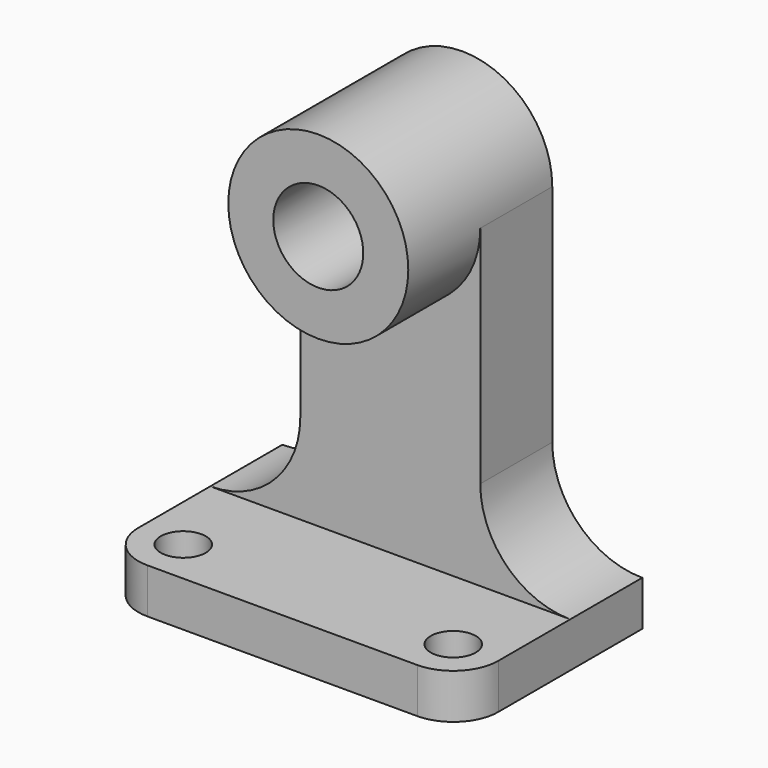
from build123d import *

# Parameters (mm, degrees)
F0_W      = 50.8
F0_H      = 63.5
F1_DEPTH  = 31.75
F2_W      = 25.4
F2_H      = 31.75
F3_DEPTH  = 19.05
F5_DEPTH  = 19.05
F6_DEPTH  = 6.35
F8_DEPTH  = 25.4
F9_DEPTH  = 25.4
F11_DEPTH = 6.35
F12_R     = 3.175
F13_DEPTH = 6.35
F14_R     = 6.35
F15_DEPTH = 25.4


# Not quite as in the source:
# - a feature names something its author has since deleted; it is built from what else it names


with BuildPart() as f1:
    # F0 (on Front) → F1 (new body)
    with BuildSketch(Plane.XZ):
        with Locations((25.4, 31.75)):
            Rectangle(F0_W, F0_H)
    extrude(amount=F1_DEPTH)

    # F2 (on face) → F3 (cut)
    with BuildSketch(Plane.XZ.offset(31.75)):
        Polygon((0, 63.5), (0, 6.35), (12.7, 6.35), (12.7, 38.1), (12.7, 63.5), align=None)
        with Locations((25.4, 22.225)):
            Rectangle(F2_W, F2_H)
        Polygon((38.1, 38.1), (38.1, 6.35), (50.8, 6.35), (50.8, 63.5), (38.1, 63.5), align=None)
    extrude(amount=-F3_DEPTH, mode=Mode.SUBTRACT)

    # F4 (on face) → F5 (cut)
    with BuildSketch(Plane.XZ.offset(31.75)):
        with BuildLine():
            ThreePointArc((12.7, 50.8), (16.4197438789, 59.7802561211), (25.4, 63.5))
            Line((25.4, 63.5), (12.7, 63.5))
            Line((12.7, 63.5), (12.7, 50.8))
        make_face()
        with BuildLine():
            ThreePointArc((25.4, 63.5), (34.3802561211, 59.7802561211), (38.1, 50.8))
            Line((38.1, 50.8), (38.1, 63.5))
            Line((38.1, 63.5), (25.4, 63.5))
        make_face()
        with BuildLine():
            Line((12.7, 38.1), (25.4, 38.1))
            ThreePointArc((25.4, 38.1), (16.4197438789, 41.8197438789), (12.7, 50.8))
            Line((12.7, 50.8), (12.7, 38.1))
        make_face()
        with BuildLine():
            Line((38.1, 38.1), (38.1, 50.8))
            ThreePointArc((38.1, 50.8), (34.3802561211, 41.8197438789), (25.4, 38.1))
            Line((25.4, 38.1), (38.1, 38.1))
        make_face()
    extrude(amount=-F5_DEPTH, mode=Mode.SUBTRACT)

    # F6 (cut): a face of the model
    f6_faces = [f1.faces().sort_by_distance(p)[0] for p in [
        (25.4, -31.75, 50.8),
    ]]
    extrude(f6_faces, amount=-F6_DEPTH, mode=Mode.SUBTRACT)

    # F7 (on face) → F8 (cut)
    with BuildSketch(Plane.XZ.offset(12.7)):
        with BuildLine():
            ThreePointArc((0, 6.35), (8.9802561211, 10.0697438789), (12.7, 19.05))
            ThreePointArc((12.7, 19.05), (8.9802561211, 28.0302561211), (0, 31.75))
            Line((0, 31.75), (0, 6.35))
        make_face()
        with BuildLine():
            Line((12.7, 50.8), (12.7, 63.5))
            Line((12.7, 63.5), (0, 63.5))
            Line((0, 63.5), (0, 31.75))
            ThreePointArc((0, 31.75), (8.9802561211, 28.0302561211), (12.7, 19.05))
            Line((12.7, 19.05), (12.7, 50.8))
        make_face()
        with BuildLine():
            Line((50.8, 63.5), (38.1, 63.5))
            Line((38.1, 63.5), (38.1, 50.8))
            Line((38.1, 50.8), (38.1, 19.0500000487))
            ThreePointArc((38.1, 19.0500000487), (41.8197438961, 28.0302561383), (50.8, 31.75))
            Line((50.8, 31.75), (50.8, 63.5))
        make_face()
        with BuildLine():
            ThreePointArc((50.8, 31.75), (41.8197438961, 28.0302561383), (38.1, 19.0500000487))
            ThreePointArc((38.1, 19.0500000487), (41.8197438617, 10.0697438961), (50.8, 6.35))
            Line((50.8, 6.35), (50.8, 31.75))
        make_face()
    extrude(amount=-F8_DEPTH, mode=Mode.SUBTRACT)

    # F9 (cut): faces of the model
    f9_faces = [f1.faces().sort_by_distance(p)[0] for p in [
        (15.5367728246, -12.7, 60.6632271754),
        (35.2632271754, -12.7, 60.6632271754),
    ]]
    extrude(f9_faces, amount=-F9_DEPTH, mode=Mode.SUBTRACT)

    # F10 (on face) → F11 (cut)
    with BuildSketch(Plane.XY.offset(6.35)):
        with BuildLine():
            Line((0, -31.75), (6.35, -31.75))
            ThreePointArc((6.35, -31.75), (1.8598719395, -29.8901280605), (0, -25.4))
            Line((0, -25.4), (0, -31.75))
        make_face()
        with BuildLine():
            Line((50.8, -31.75), (50.8, -25.4))
            ThreePointArc((50.8, -25.4), (48.9401280605, -29.8901280605), (44.45, -31.75))
            Line((44.45, -31.75), (50.8, -31.75))
        make_face()
    extrude(amount=-F11_DEPTH, mode=Mode.SUBTRACT)

    # F12 (on face) → F13 (cut)
    with BuildSketch(Plane.XY.offset(6.35)):
        with Locations((6.35, -25.4)):
            Circle(F12_R)
        with Locations((44.45, -25.4)):
            Circle(F12_R)
    extrude(amount=-F13_DEPTH, mode=Mode.SUBTRACT)

    # F14 (on face) → F15 (cut)
    with BuildSketch(Plane(origin=(0, 0, 0), x_dir=(-1, 0, 0), z_dir=(0, 1, 0))):
        with Locations((-25.4, 50.8)):
            Circle(F14_R)
    extrude(amount=-F15_DEPTH, mode=Mode.SUBTRACT)


solid = f1.part
